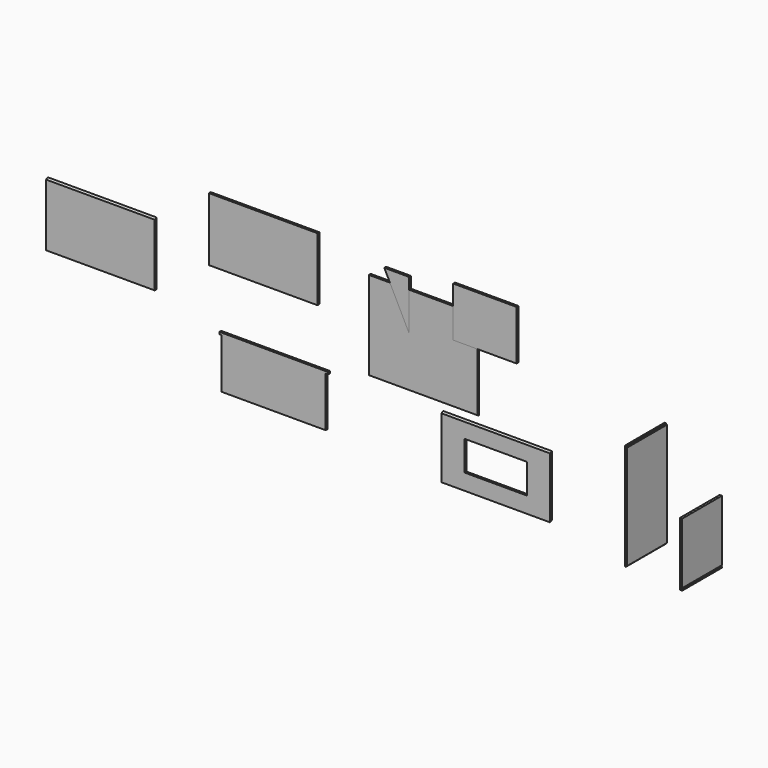
from build123d import *

# Parameters (mm, degrees)
F0_W      = 152.4
F0_H      = 86.7664
F0_W_2    = 87.2998
F0_H_2    = 41.7068
F1_DEPTH  = 3.175
F2_W      = 152.4
F2_H      = 125.4125
F3_DEPTH  = 3.175
F5_DEPTH  = 3.175
F6_W      = 152.4
F6_H      = 88.9
F7_DEPTH  = 3.175
F9_DEPTH  = 3.175
F10_W     = 88.9
F10_H     = 69.85
F11_DEPTH = 3.175
F12_SIZE2 = 1.518471
F12_SIZE  = 3.17499
F13_SIZE2 = 1.58714
F13_SIZE  = 3.17499
F14_W     = 152.4
F14_H     = 88.9
F15_DEPTH = 3.175
F16_SIZE2 = 1.58714
F16_SIZE  = 3.17499
F17_SIZE2 = 1.58714
F17_SIZE  = 3.17499
F19_DEPTH = 69.85
F21_DEPTH = 69.85


# Not quite as in the source:
# - a fillet or chamfer is up to 0.001 mm smaller than in the source, because OpenCascade refuses the exact size


with BuildPart() as f1:
    # F0 (on Front) → F1 (new body)
    with BuildSketch(Plane.XZ):
        with Locations((48.9966, -30.7150018784)):
            Rectangle(F0_W, F0_H)
        with Locations((48.9966, -30.7150018784)):
            Rectangle(F0_W_2, F0_H_2, mode=Mode.SUBTRACT)
    extrude(amount=F1_DEPTH)

    # F12 (size 3.175 and 1.5184806323 in the source; OpenCascade refuses exactly that, so slightly less here)
    f12_edges = [f1.edges().sort_by_distance(p)[0] for p in [
        (48.9966, 0, -74.098202),
    ]]
    f12_side = f1.faces().sort_by_distance((48.9966, -1.5875, -74.098202))[0]
    chamfer(f12_edges, length=F12_SIZE, length2=F12_SIZE2, reference=f12_side)

    # F13 (size 3.175 and 1.5871501317 in the source; OpenCascade refuses exactly that, so slightly less here)
    f13_edges = [f1.edges().sort_by_distance(p)[0] for p in [
        (48.9966, -3.175, 12.668198),
    ]]
    f13_side = f1.faces().sort_by_distance((48.9966, -1.5875, 12.668198))[0]
    chamfer(f13_edges, length=F13_SIZE, length2=F13_SIZE2, reference=f13_side)


with BuildPart() as f3:
    # F2 (on Front) → F3 (new body)
    with BuildSketch(Plane.XZ):
        with Locations((-52.8449798107, 86.1903589696)):
            Rectangle(F2_W, F2_H)
    extrude(amount=F3_DEPTH)

    # F17 (size 3.175 and 1.5871501317 in the source; OpenCascade refuses exactly that, so slightly less here)
    f17_edges = [f3.edges().sort_by_distance(p)[0] for p in [
        (-52.84498, -3.175, 23.484109),
    ]]
    f17_side = f3.faces().sort_by_distance((-52.84498, -1.5875, 23.484109))[0]
    chamfer(f17_edges, length=F17_SIZE, length2=F17_SIZE2, reference=f17_side)


with BuildPart() as f5:
    # F4 (on Front) → F5 (new body)
    with BuildSketch(Plane.XZ):
        Polygon((-335.5122112751, -62.6780449331), (-189.4622112751, -62.6780449331), (-189.4622112751, 7.1719550669), (-186.2872112751, 7.1719550669), (-186.2872112751, 10.3469550669), (-338.6872112751, 10.3469550669), (-338.6872112751, 7.1719550669), (-335.5122112751, 7.1719550669), align=None)
    extrude(amount=F5_DEPTH)


with BuildPart() as f7:
    # F6 (on Front) → F7 (new body)
    with BuildSketch(Plane.XZ):
        with Locations((-277.1691465855, 132.4105263472)):
            Rectangle(F6_W, F6_H)
    extrude(amount=F7_DEPTH)


with BuildPart() as f9:
    # F8 (on Front) → F9 (new body)
    with BuildSketch(Plane.XZ):
        Polygon((-107.2789654136, 164.7035479546), (-72.3539654136, 94.8535479546), (-72.3539654136, 164.7035479546), align=None)
    extrude(amount=F9_DEPTH)


with BuildPart() as f11:
    # F10 (on Front) → F11 (new body)
    with BuildSketch(Plane.XZ):
        with Locations((33.8623570919, 141.7346980453)):
            Rectangle(F10_W, F10_H)
    extrude(amount=F11_DEPTH)


with BuildPart() as f15:
    # F14 (on Front) → F15 (new body)
    with BuildSketch(Plane.XZ):
        with Locations((-505.4994225502, 76.4577066326)):
            Rectangle(F14_W, F14_H)
    extrude(amount=F15_DEPTH)

    # F16 (size 3.175 and 1.5871501317 in the source; OpenCascade refuses exactly that, so slightly less here)
    f16_edges = [f15.edges().sort_by_distance(p)[0] for p in [
        (-505.499423, -3.175, 120.907707),
    ]]
    f16_side = f15.faces().sort_by_distance((-505.499423, -1.5875, 120.907707))[0]
    chamfer(f16_edges, length=F16_SIZE, length2=F16_SIZE2, reference=f16_side)


with BuildPart() as f19:
    # F18 (on Front) → F19 (new body)
    with BuildSketch(Plane.XZ):
        Polygon((363.7785966866, 35.07166363), (360.6035966866, 35.07166363), (360.6035966866, -53.82833637), (363.7785966866, -53.82833637), (363.7785966866, -52.24083637), (362.1910966866, -52.24083637), (362.1910966866, -50.65333637), (363.7785966866, -50.65333637), align=None)
    extrude(amount=F19_DEPTH)


with BuildPart() as f21:
    # F20 (on Front) → F21 (new body)
    with BuildSketch(Plane.XZ):
        Polygon((284.9999441053, 97.662555486), (284.9999441053, 99.250055486), (283.4124441053, 99.250055486), (283.4124441053, -49.974944514), (284.9999441053, -49.974944514), (284.9999441053, -48.387444514), (286.5874441053, -48.387444514), (286.5874441053, 97.662555486), align=None)
    extrude(amount=F21_DEPTH)


solid = Compound([f1.part, f3.part, f5.part, f7.part, f9.part, f11.part, f15.part, f19.part, f21.part])
